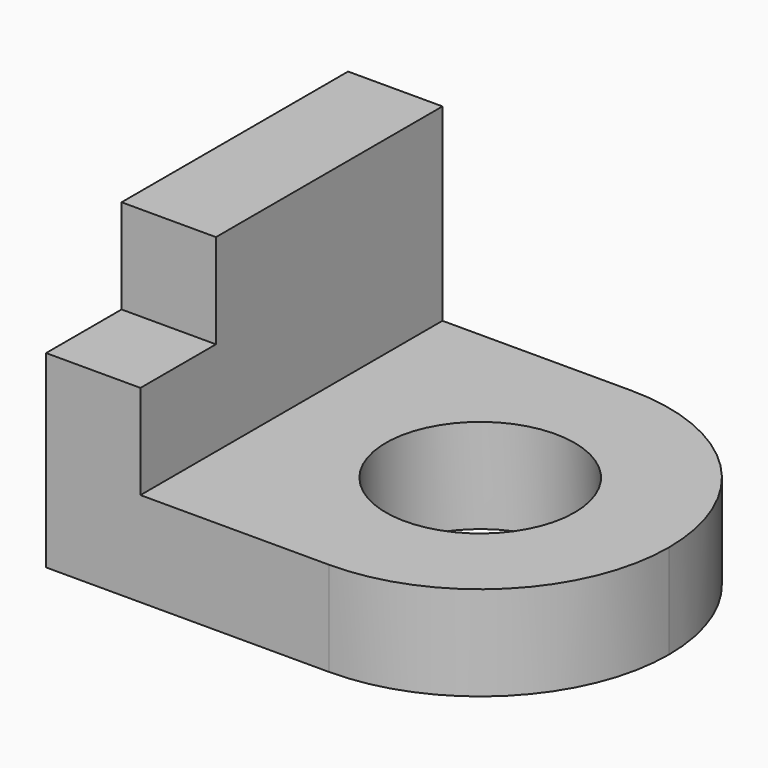
from build123d import *

# Parameters (mm, degrees)
F1_DEPTH = 20
F2_R     = 19.99999
F3_R     = 10
F4_DEPTH = 10
F5_W     = 10
F5_H     = 10
F6_DEPTH = 10


# Not quite as in the source:
# - a fillet or chamfer is up to 0.001 mm smaller than in the source, because OpenCascade refuses the exact size


with BuildPart() as f1:
    # F0 (on Front) → F1 (new body, symmetric)
    with BuildSketch(Plane.XZ):
        Polygon((0, 30), (0, 0), (50, 0), (50, 10), (10, 10), (10, 30), align=None)
    extrude(amount=F1_DEPTH, both=True)

    # F2 (radius 20 in the source; OpenCascade refuses exactly that, so slightly less here)
    f2_edges = [f1.edges().sort_by_distance(p)[0] for p in [
        (50, -20, 5),
        (50, 20, 5),
    ]]
    fillet(f2_edges, radius=F2_R)

    # F3 (on face) → F4 (cut, through all)
    with BuildSketch(Plane.XY.offset(10)):
        with Locations((30, 0)):
            Circle(F3_R)
    extrude(amount=-F4_DEPTH, mode=Mode.SUBTRACT)

    # F5 (on face) → F6 (cut, through all)
    with BuildSketch(Plane.YZ.offset(10)):
        with Locations((-15, 25)):
            Rectangle(F5_W, F5_H)
    extrude(amount=-F6_DEPTH, mode=Mode.SUBTRACT)


solid = f1.part
